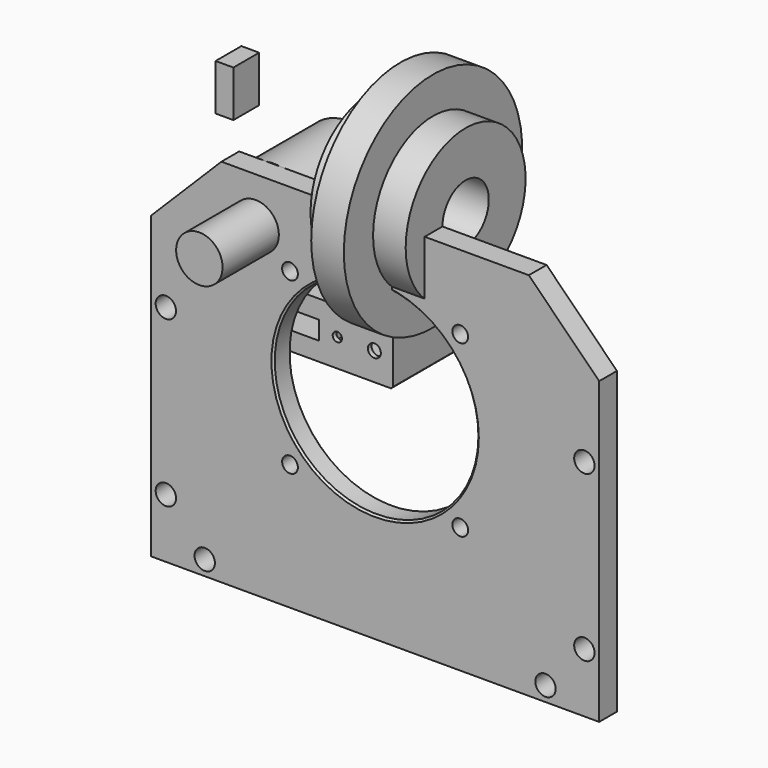
from build123d import *

# Parameters (mm, degrees)
F0_W           = 120
F0_H           = 30
F1_DEPTH       = 25
F2_W           = 120
F2_H           = 30
F2_W_2         = 40
F2_H_2         = 10
F3_DEPTH       = 25
F4_T           = -2.5
F6_D           = 5
F7_D           = 7
F8_SIZE        = 1
F9_R           = 25
F9_R_2         = 12.5
F10_DEPTH      = 50
F13_R          = 12.5366828167
F14_DEPTH      = 50
F14_DEPTH_BACK = 50
F15_W          = 242
F15_H          = 200
F15_R          = 55
F16_DEPTH      = 12
F17_SIZE       = 38
F19_D          = 8.5
F21_D          = 11
F22_SIZE       = 1
F23_W          = 9.6032470465
F23_H          = 17.4058834091
F24_DEPTH      = 25


with BuildPart() as f1:
    # F0 (on Front) → F1 (new body)
    with BuildSketch(Plane.XZ):
        with Locations((-60, 15)):
            Rectangle(F0_W, F0_H)
    extrude(amount=F1_DEPTH)

    # F2 (on face) → F3 (join)
    with BuildSketch(Plane.XZ.offset(25)):
        with Locations((-60, 15)):
            Rectangle(F2_W, F2_H)
        with Locations((-60, 15)):
            Rectangle(F2_W_2, F2_H_2, mode=Mode.SUBTRACT)
    extrude(amount=F3_DEPTH)

    # F4
    f4_openings = [f1.faces().sort_by_distance(p)[0] for p in [
        (-60, 0, 15),
    ]]
    offset(amount=F4_T, openings=f4_openings, kind=Kind.INTERSECTION)

    # F6 (through all)
    with Locations(Plane.XZ.offset(50)):
        with Locations((-90, 15), (-30, 15)):
            Hole(F6_D / 2)

    # F7 (through all)
    with Locations(Plane.XZ.offset(50)):
        with Locations((-10, 15)):
            Hole(F7_D / 2)

    # F8
    f8_edges = [f1.edges().sort_by_distance(p)[0] for p in [
        (-120, -25, 30),
        (-120, -25, 0),
        (0, -25, 30),
        (0, -25, 0),
    ]]
    chamfer(f8_edges, length=F8_SIZE)


with BuildPart() as f10:
    # F9 (on Front) → F10 (new body)
    with BuildSketch(Plane.XZ):
        with Locations((-64.5213648677, 61.3059587777)):
            Circle(F9_R)
        with Locations((-64.5213648677, 61.3059587777)):
            Circle(F9_R_2, mode=Mode.SUBTRACT)
    extrude(amount=F10_DEPTH)


with BuildPart() as f14:
    # F13 (on offset) → F14 (new body, two sides)
    with BuildSketch(Plane.XZ.offset(50)) as f14_sk:
        with Locations((-64.5213648677, 61.3059587777)):
            Circle(F13_R)
    extrude(amount=-F14_DEPTH)
    extrude(f14_sk.sketch, amount=F14_DEPTH_BACK)


with BuildPart() as f16:
    # F15 (on offset) → F16 (new body)
    with BuildSketch(Plane.XZ.offset(50)):
        with Locations((0, -14)):
            Rectangle(F15_W, F15_H)
        Circle(F15_R, mode=Mode.SUBTRACT)
    extrude(amount=F16_DEPTH)

    # F17
    f17_edges = [f16.edges().sort_by_distance(p)[0] for p in [
        (-121, -56, 86),
        (121, -56, 86),
    ]]
    chamfer(f17_edges, length=F17_SIZE)

    # F19 (through all)
    with Locations(Plane.XZ.offset(62)):
        with Locations((-45.9619407771, 45.9619407771), (45.9619407771, 45.9619407771), (45.9619407771, -45.9619407771), (-45.9619407771, -45.9619407771)):
            Hole(F19_D / 2)

    # F21 (through all)
    with Locations(Plane.XZ.offset(62)):
        with Locations((-113, 7), (113, 7), (113, -82), (92, -106), (-92, -106), (-113, -82)):
            Hole(F21_D / 2)

    # F22
    f22_edges = [f16.edges().sort_by_distance(p)[0] for p in [
        (-55, -62, 0),
        (-55, -50, 0),
    ]]
    chamfer(f22_edges, length=F22_SIZE)


with BuildPart() as f24:
    # F23 (on face) → F24 (new body)
    with BuildSketch(Plane.XY.offset(86)):
        with Locations((-107.555270195, -20.5133124255)):
            Rectangle(F23_W, F23_H)
    extrude(amount=F24_DEPTH)


with BuildPart() as f26:
    # F25 (on face) → F26 (revolve)
    with BuildSketch(Plane.XY.offset(86)):
        Polygon((26.7714690417, -50), (-24.6196500957, -50), (-24.6196500957, -74.833586812), (-8.4409639239, -74.833586812), (-8.4409639239, -94.581104815), (9.1652534902, -94.581104815), (9.1652534902, -74.833586812), (26.7714690417, -74.833586812), align=None)
    revolve(axis=Axis((1.0507404804, -34.3671105802, 86), (1, 0, 0)))


solid = Compound([f1.part, f10.part, f14.part, f16.part, f24.part, f26.part])
